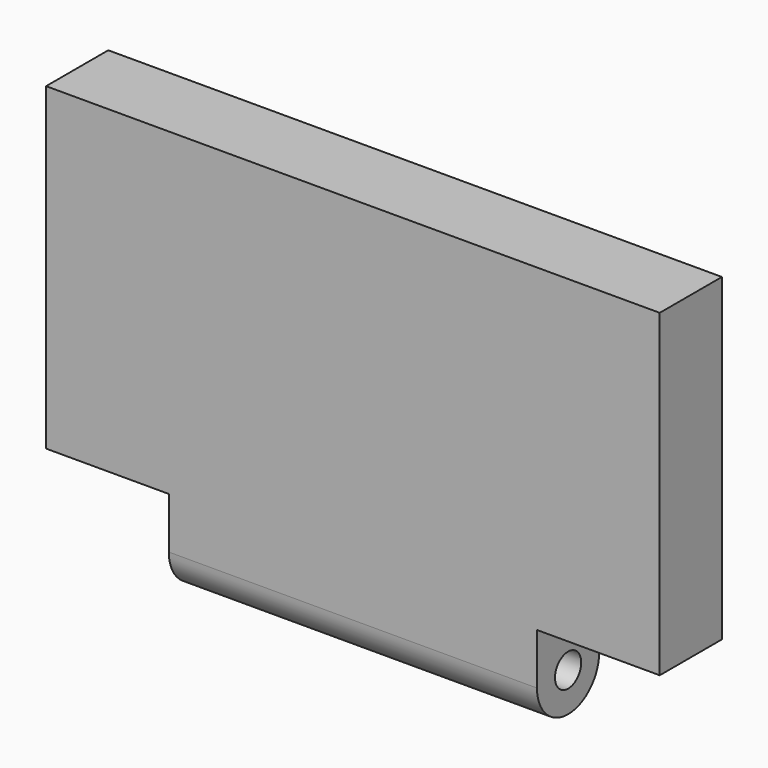
from build123d import *

# Parameters (mm, degrees)
F1_DEPTH = 19
F2_R     = 4
F3_DEPTH = 120.001
F4_R     = 9.49999


# Not quite as in the source:
# - a fillet or chamfer is up to 0.001 mm smaller than in the source, because OpenCascade refuses the exact size


with BuildPart() as f1:
    # F0 (on Front) → F1 (new body)
    with BuildSketch(Plane.XZ):
        Polygon((-45, -50), (45, -50), (45, -28), (75, -28), (75, 50), (-75, 50), (-75, -28), (-45, -28), align=None)
    extrude(amount=F1_DEPTH)

    # F2 (on face) → F3 (cut, through all)
    with BuildSketch(Plane(origin=(-45, 0, 0), x_dir=(0, -1, 0), z_dir=(-1, 0, 0))):
        with Locations((9.5, -40.5)):
            Circle(F2_R)
    extrude(amount=-F3_DEPTH, mode=Mode.SUBTRACT)

    # F4 (radius 9.5 in the source; OpenCascade refuses exactly that, so slightly less here)
    f4_edges = [f1.edges().sort_by_distance(p)[0] for p in [
        (0, 0, -50),
        (0, -19, -50),
    ]]
    fillet(f4_edges, radius=F4_R)


solid = f1.part
